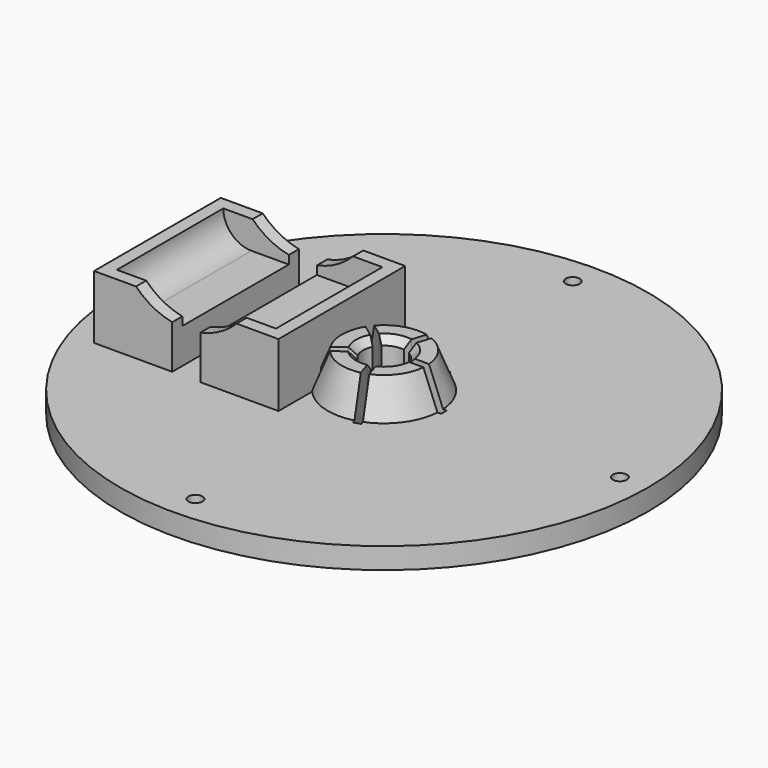
from build123d import *

# Parameters (mm, degrees)
F0_R      = 37.5
F0_R_2    = 1
F0_R_3    = 3
F1_DEPTH  = 3
F2_R      = 8
F2_R_2    = 3
F3_DEPTH  = 5
F4_SIZE2  = 4.99999
F4_SIZE   = 1.99999
F5_SIZE   = 1
F7_DEPTH  = 8.001
F8_R      = 1.5
F9_DEPTH  = 3.001
F10_W     = 26.2
F10_H     = 22.5
F11_DEPTH = 9
F12_W     = 22.6
F12_H     = 18.9
F13_DEPTH = 4
F14_R     = 3.99999
F15_W     = 4
F15_H     = 22.5
F16_DEPTH = 9
F18_DEPTH = 25


# Not quite as in the source:
# - a fillet or chamfer is up to 0.001 mm smaller than in the source, because OpenCascade refuses the exact size


with BuildPart() as f1:
    # F0 (on Top) → F1 (new body)
    with BuildSketch(Plane.XY):
        Circle(F0_R)
        with Locations((0, -33.5)):
            Circle(F0_R_2, mode=Mode.SUBTRACT)
        with Locations((-33.5, 0)):
            Circle(F0_R_2, mode=Mode.SUBTRACT)
        Circle(F0_R_3, mode=Mode.SUBTRACT)
        with Locations((33.5, 0)):
            Circle(F0_R_2, mode=Mode.SUBTRACT)
        with Locations((0, 33.5)):
            Circle(F0_R_2, mode=Mode.SUBTRACT)
    extrude(amount=F1_DEPTH)

    # F2 (on face) → F3 (join)
    with BuildSketch(Plane.XY.offset(3)):
        Circle(F2_R)
        Circle(F2_R_2, mode=Mode.SUBTRACT)
    extrude(amount=F3_DEPTH)

    # F4 (size 2 and 5 in the source; OpenCascade refuses exactly that, so slightly less here)
    f4_edges = [f1.edges().sort_by_distance(p)[0] for p in [
        (-8, 0, 8),
    ]]
    f4_side = f1.faces().sort_by_distance((-7.773726, 0, 8))[0]
    chamfer(f4_edges, length=F4_SIZE, length2=F4_SIZE2, reference=f4_side)

    # F5
    f5_edges = [f1.edges().sort_by_distance(p)[0] for p in [
        (-3, 0, 0),
        (3, 0, 4),
        (-3, 0, 8),
    ]]
    chamfer(f5_edges, length=F5_SIZE)

    # F6 (on face) → F7 (cut, through all)
    with BuildSketch(Plane(origin=(0, 0, 0), x_dir=(1, 0, 0), z_dir=(0, 0, -1))):
        with BuildLine():
            Line((-1.7286498598, 1.8739716279), (-2.9167940342, 2.7372089))
            ThreePointArc((-2.9167940342, 2.7372089), (-3.2360679775, 2.3511410092), (-3.5045792865, 1.9281919056))
            Line((-3.5045792865, 1.9281919056), (-2.3164351121, 1.0649546335))
            Line((-2.3164351121, 1.0649546335), (-1.7286498598, 1.8739716279))
        make_face()
        with BuildLine():
            Line((1.2480707441, 2.2231327936), (1.7019014352, 3.6198800401))
            ThreePointArc((1.7019014352, 3.6198800401), (1.2360679775, 3.8042260652), (0.7508449189, 3.9288970345))
            Line((0.7508449189, 3.9288970345), (0.2970142278, 2.5321497879))
            Line((0.2970142278, 2.5321497879), (1.2480707441, 2.2231327936))
        make_face()
        with BuildLine():
            ThreePointArc((0.7508449189, 3.9288970345), (1.2360679775, 3.8042260652), (1.7019014352, 3.6198800401))
            Line((1.7019014352, 3.6198800401), (3.1021727103, 7.9294718913))
            Line((3.1021727103, 7.9294718913), (2.151116194, 8.2384888857))
            Line((2.151116194, 8.2384888857), (0.7508449189, 3.9288970345))
        make_face()
        with BuildLine():
            Line((8.5, -0.5), (8.5, 0.5))
            Line((8.5, 0.5), (3.9686269666, 0.5))
            ThreePointArc((3.9686269666, 0.5), (3.9921490369, 0.2504916502), (4, 0))
            ThreePointArc((4, 0), (3.9921490369, -0.2504916502), (3.9686269666, -0.5))
            Line((3.9686269666, -0.5), (8.5, -0.5))
        make_face()
        with BuildLine():
            Line((3.1021727103, -7.9294718913), (1.7019014352, -3.6198800401))
            ThreePointArc((1.7019014352, -3.6198800401), (1.2360679775, -3.8042260652), (0.7508449189, -3.9288970345))
            Line((0.7508449189, -3.9288970345), (2.151116194, -8.2384888857))
            Line((2.151116194, -8.2384888857), (3.1021727103, -7.9294718913))
        make_face()
        with BuildLine():
            ThreePointArc((4, 0), (3.9921490369, 0.2504916502), (3.9686269666, 0.5))
            Line((3.9686269666, 0.5), (2.5, 0.5))
            Line((2.5, 0.5), (2.5, -0.5))
            Line((2.5, -0.5), (3.9686269666, -0.5))
            ThreePointArc((3.9686269666, -0.5), (3.9921490369, -0.2504916502), (4, 0))
        make_face()
        with BuildLine():
            ThreePointArc((0.7508449189, -3.9288970345), (1.2360679775, -3.8042260652), (1.7019014352, -3.6198800401))
            Line((1.7019014352, -3.6198800401), (1.2480707441, -2.2231327936))
            Line((1.2480707441, -2.2231327936), (0.2970142278, -2.5321497879))
            Line((0.2970142278, -2.5321497879), (0.7508449189, -3.9288970345))
        make_face()
        with BuildLine():
            Line((-6.582751826, -5.4006831417), (-2.9167940342, -2.7372089))
            ThreePointArc((-2.9167940342, -2.7372089), (-3.2360679775, -2.3511410092), (-3.5045792865, -1.9281919056))
            Line((-3.5045792865, -1.9281919056), (-7.1705370783, -4.5916661473))
            Line((-7.1705370783, -4.5916661473), (-6.582751826, -5.4006831417))
        make_face()
        with BuildLine():
            ThreePointArc((-3.5045792865, -1.9281919056), (-3.2360679775, -2.3511410092), (-2.9167940342, -2.7372089))
            Line((-2.9167940342, -2.7372089), (-1.7286498598, -1.8739716279))
            Line((-1.7286498598, -1.8739716279), (-2.3164351121, -1.0649546335))
            Line((-2.3164351121, -1.0649546335), (-3.5045792865, -1.9281919056))
        make_face()
        with BuildLine():
            ThreePointArc((-3.5045792865, 1.9281919056), (-3.2360679775, 2.3511410092), (-2.9167940342, 2.7372089))
            Line((-2.9167940342, 2.7372089), (-6.582751826, 5.4006831417))
            Line((-6.582751826, 5.4006831417), (-7.1705370783, 4.5916661473))
            Line((-7.1705370783, 4.5916661473), (-3.5045792865, 1.9281919056))
        make_face()
    extrude(amount=-F7_DEPTH, mode=Mode.SUBTRACT)

    # F8 (on face) → F9 (cut, through all)
    with BuildSketch(Plane.XY.offset(3)):
        with Locations((-19.1, 3)):
            Circle(F8_R)
        with Locations((-19.1, -3)):
            Circle(F8_R)
    extrude(amount=-F9_DEPTH, mode=Mode.SUBTRACT)

    # F10 (on face) → F11 (join)
    with BuildSketch(Plane.XY.offset(3)):
        with Locations((-19.1, 0)):
            Rectangle(F10_W, F10_H)
    extrude(amount=F11_DEPTH)

    # F12 (on face) → F13 (cut)
    with BuildSketch(Plane.XY.offset(12)):
        with Locations((-19.1, 0)):
            Rectangle(F12_W, F12_H)
    extrude(amount=-F13_DEPTH, mode=Mode.SUBTRACT)

    # F14 (radius 4 in the source; OpenCascade refuses exactly that, so slightly less here)
    f14_edges = [f1.edges().sort_by_distance(p)[0] for p in [
        (-30.4, 0, 8),
        (-7.8, 0, 8),
    ]]
    fillet(f14_edges, radius=F14_R)

    # F15 (on face) → F16 (cut, through all)
    with BuildSketch(Plane.XY.offset(12)):
        with Locations((-19.1, 0)):
            Rectangle(F15_W, F15_H)
    extrude(amount=-F16_DEPTH, mode=Mode.SUBTRACT)

    # F17 (on face) → F18 (cut, symmetric)
    with BuildSketch(Plane.XZ.offset(-9.45)):
        with BuildLine():
            ThreePointArc((-11.9585715715, 12), (-9.8421848073, 15.2194103823), (-9.1, 19))
            ThreePointArc((-9.1, 19), (-26.8459666924, 25.3245553203), (-17.1, 9.2020410289))
            Line((-17.1, 9.2020410289), (-17.1, 12))
            Line((-17.1, 12), (-11.9585715715, 12))
        make_face()
        with BuildLine():
            Line((-17.1, 12), (-17.1, 9.2020410289))
            ThreePointArc((-17.1, 9.2020410289), (-14.3199820053, 10.2164114412), (-11.9585715715, 12))
            Line((-11.9585715715, 12), (-17.1, 12))
        make_face()
    extrude(amount=F18_DEPTH, both=True, mode=Mode.SUBTRACT)


solid = f1.part
